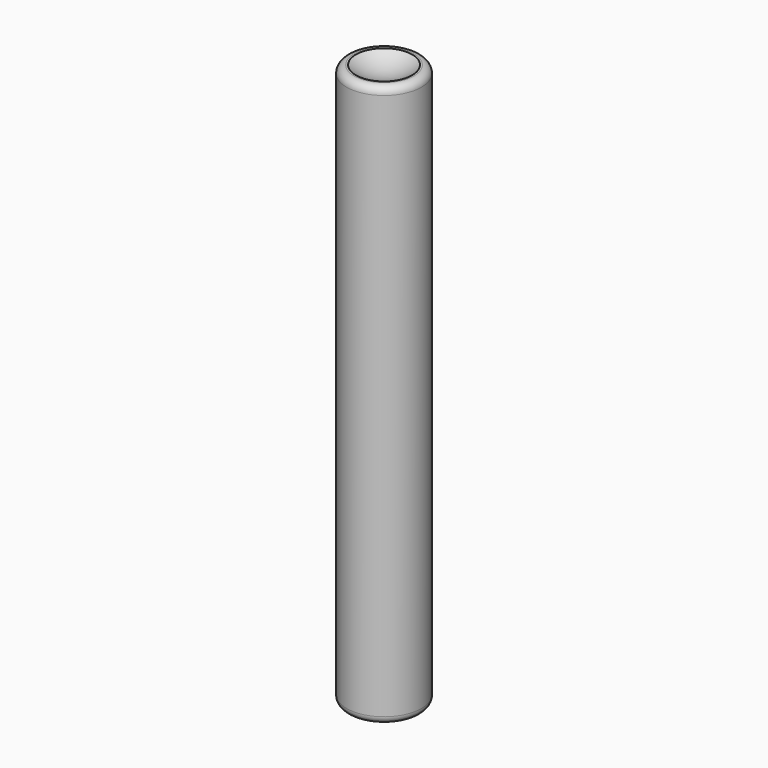
from build123d import *

# Parameters (mm, degrees)
F0_R          = 4
F1_DEPTH      = 30
F1_DEPTH_BACK = 30
F4_R          = 0.8
F6_START      = -1.5
F5_R          = 3
F6_DEPTH      = 13.1


# Not quite as in the source:
# - a pattern or mirror of a feature is missing from the dataset's text; its kind, count and spacing are read off the source's solid


with BuildPart() as f1:
    # F0 (on Top) → F1 (new body, two sides)
    with BuildSketch(Plane.XY) as f1_sk:
        Circle(F0_R)
    extrude(amount=F1_DEPTH)
    extrude(f1_sk.sketch, amount=-F1_DEPTH_BACK)

    # F2 (on Front) → F3 (revolve, cut)
    with BuildSketch(Plane.XZ):
        with BuildLine():
            Line((0, 34), (0, 29))
            ThreePointArc((0, 29), (3.5355339059, 30.4644660941), (5, 34))
            ThreePointArc((5, 34), (3.5355339059, 37.5355339059), (0, 39))
            Line((0, 39), (0, 34))
        make_face()
    f3 = revolve(axis=Axis((0, 0, 36.5), (0, 0, -1)), mode=Mode.SUBTRACT)

    # F3_copies: F3 across plane
    add(f3.mirror(Plane(origin=(0, 0, 0), x_dir=(-1, 0, 0), z_dir=(0, 0, -1))), mode=Mode.SUBTRACT)

    # F4
    f4_edges = [f1.edges().sort_by_distance(p)[0] for p in [
        (-4, 0, 30),
        (-4, 0, -30),
    ]]
    fillet(f4_edges, radius=F4_R)

    # F5 (on face) → F6 (cut)
    with BuildSketch(Plane.XY.offset(30).offset(F6_START)):
        Circle(F5_R)
    f6 = extrude(amount=-F6_DEPTH, mode=Mode.SUBTRACT)

    # F6_copies: F6 across plane
    add(f6.mirror(Plane(origin=(0, 0, 0), x_dir=(-1, 0, 0), z_dir=(0, 0, -1))), mode=Mode.SUBTRACT)


solid = f1.part
